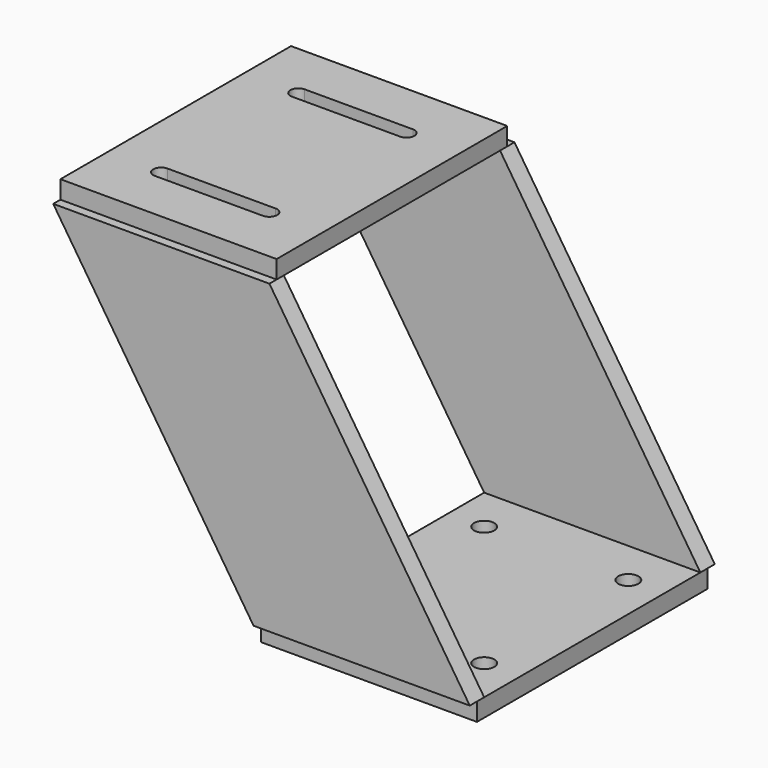
from build123d import *

# Parameters (mm, degrees)
F0_W      = 152.4
F0_H      = 203.2
F1_DEPTH  = 12.7
F3_D      = 14.2875
F5_W      = 152.4
F5_H      = 203.2
F6_DEPTH  = 12.7
F8_DEPTH  = 241.301
F10_DEPTH = 6.35


# Not quite as in the source:
# - a length typed as a fraction of an inch, garbled in the dataset ("3 / 203.2 mm" for 3/8 in), is restored


with BuildPart() as f1:
    # F0 (on Top) → F1 (new body)
    with BuildSketch(Plane.XY):
        Rectangle(F0_W, F0_H)
    extrude(amount=F1_DEPTH)

    # F3 (through all)
    with Locations(Plane.XY.offset(12.7)):
        with Locations((-50.8, 63.5), (50.8, 63.5), (-50.8, -63.5), (50.8, -63.5)):
            Hole(F3_D / 2)


with BuildPart() as f6:
    # F5 (on offset) → F6 (new body)
    with BuildSketch(Plane(origin=(0, 0, 241.3), x_dir=(1, 0, 0), z_dir=(0, 0, -1))):
        with Locations((-141.224, 0)):
            Rectangle(F5_W, F5_H)
    extrude(amount=F6_DEPTH)

    # F7 (on face) → F8 (cut, through all)
    with BuildSketch(Plane.XY.offset(241.3)):
        with BuildLine():
            ThreePointArc((-179.324, -54.864), (-184.912, -60.452), (-179.324, -66.04))
            Line((-179.324, -66.04), (-103.124, -66.04))
            ThreePointArc((-103.124, -66.04), (-97.536, -60.452), (-103.124, -54.864))
            Line((-103.124, -54.864), (-179.324, -54.864))
        make_face()
        with BuildLine():
            Line((-179.324, 54.864), (-103.124, 54.864))
            ThreePointArc((-103.124, 54.864), (-97.536, 60.452), (-103.124, 66.04))
            Line((-103.124, 66.04), (-179.324, 66.04))
            ThreePointArc((-179.324, 66.04), (-184.912, 60.452), (-179.324, 54.864))
        make_face()
    extrude(amount=-F8_DEPTH, mode=Mode.SUBTRACT)


with BuildPart() as f10:
    # F9 (on face) → F10 (new body, symmetric)
    with BuildSketch(Plane.XZ.offset(101.6)):
        Polygon((-65.024, 228.6), (-217.424, 228.6), (-76.2, 12.7), (76.2, 12.7), align=None)
    extrude(amount=F10_DEPTH, both=True)


with BuildPart() as f11_1:
    # F11: instance of F10
    add(f10.part.mirror(Plane.XZ))


solid = Compound([f1.part, f6.part, f10.part, f11_1.part])
